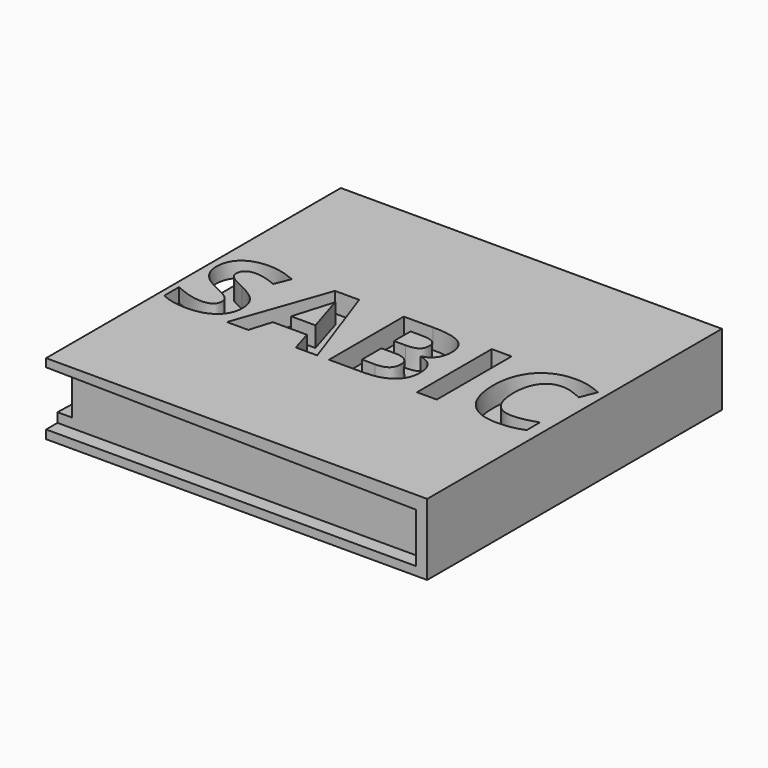
from build123d import *

# Parameters (mm, degrees)
F0_W         = 63.4120106697
F0_H         = 128.9969310164
F0_W_2       = 70.033095777
F1_DEPTH     = 25
F2_TEXT_SIZE = 45.8475779074
F3_DEPTH     = 7
F6_DEPTH     = 5
F7_W         = 125.2561286092
F7_H         = 17.6452279557
F8_DEPTH     = 5
F10_DEPTH    = 5


# Not quite as in the source:
# - Text() gives the source's letters only with a copy of the font that has no kerning and outlines rounded to 1/6400 em; it was checked with that copy


with BuildPart() as f1:
    # F0 (on Top) → F1 (new body)
    with BuildSketch(Plane.XY):
        with Locations((31.7060053349, -0.8814968169)):
            Rectangle(F0_W, F0_H)
        with Locations((-35.0165478885, -0.8814968169)):
            Rectangle(F0_W_2, F0_H)
    extrude(amount=F1_DEPTH)

    # F2 (on face) → F3 (cut)
    with BuildSketch(Plane.XY.offset(25)):
        with Locations((-70.033095777, -17.8130346296)):
            Text('SABIC', F2_TEXT_SIZE, font='Open Sans', font_style=FontStyle.BOLD, text_align=(TextAlign.LEFT, TextAlign.BOTTOM))
    extrude(amount=-F3_DEPTH, mode=Mode.SUBTRACT)

    # F5 (on face) → F6 (cut)
    with BuildSketch(Plane.XZ.offset(65.3799623251)):
        Polygon((59.5022104681, 20.4024482518), (-70.033095777, 22.1620090306), (-70.033095777, 3.0089574866), (59.5022104681, 3.0089574866), align=None)
    extrude(amount=-F6_DEPTH, mode=Mode.SUBTRACT)

    # F7 (on face) → F8 (cut)
    with BuildSketch(Plane(origin=(0, 63.6169686913, 0), x_dir=(-1, 0, 0), z_dir=(0, 1, 0))):
        with Locations((7.4050314724, 11.4375728881)):
            Rectangle(F7_W, F7_H)
    extrude(amount=-F8_DEPTH, mode=Mode.SUBTRACT)

    # F9 (on face) → F10 (cut)
    with BuildSketch(Plane(origin=(-70.033095777, 0, 0), x_dir=(0, -1, 0), z_dir=(-1, 0, 0))):
        Polygon((60.419537127, 21.1907289922), (-57.1432411671, 18.6217240989), (-57.1432411671, 3.7280179095), (60.419537127, 6.2970228028), align=None)
    extrude(amount=-F10_DEPTH, mode=Mode.SUBTRACT)


solid = f1.part
